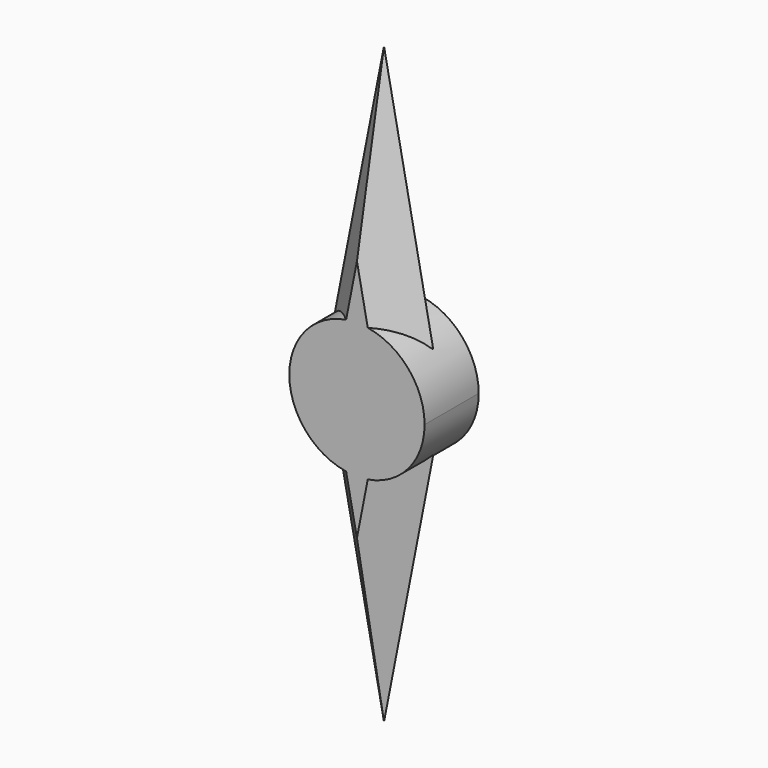
from build123d import *

# Parameters (mm, degrees)
F1_DEPTH = 12.7
F2_SIZE  = 6.34999


# Not quite as in the source:
# - a fillet or chamfer is up to 0.001 mm smaller than in the source, because OpenCascade refuses the exact size


with BuildPart() as f1:
    # F0 (on Front) → F1 (new body)
    with BuildSketch(Plane.XZ):
        with BuildLine():
            Line((0, 0), (12.7, 0))
            ThreePointArc((12.7, 0), (11.8071097568, 4.6778370206), (9.2539906785, 8.6979110436))
            ThreePointArc((9.2539906785, 8.6979110436), (5.0411570967, 11.6566176538), (0, 12.7))
            Line((0, 12.7), (0, 0))
        make_face()
        with BuildLine():
            ThreePointArc((9.2539906785, -8.6979110436), (11.8071097568, -4.6778370206), (12.7, 0))
            Line((12.7, 0), (0, 0))
            Line((0, 0), (0, -12.7))
            ThreePointArc((0, -12.7), (5.0411570967, -11.6566176538), (9.2539906785, -8.6979110436))
        make_face()
        with BuildLine():
            ThreePointArc((0, 12.7), (5.0411570967, 11.6566176538), (9.2539906785, 8.6979110436))
            Line((9.2539906785, 8.6979110436), (0, 55.8542348444))
            Line((0, 55.8542348444), (-9.2539906785, 8.6979110436))
            ThreePointArc((-9.2539906785, 8.6979110436), (-5.0411570967, 11.6566176538), (0, 12.7))
        make_face()
        with BuildLine():
            Line((0, -55.8542348444), (9.2539906785, -8.6979110436))
            ThreePointArc((9.2539906785, -8.6979110436), (5.0411570967, -11.6566176538), (0, -12.7))
            ThreePointArc((0, -12.7), (-5.0411570967, -11.6566176538), (-9.2539906785, -8.6979110436))
            Line((-9.2539906785, -8.6979110436), (0, -55.8542348444))
        make_face()
        with BuildLine():
            Line((-12.7, 0), (0, 0))
            Line((0, 0), (0, 12.7))
            ThreePointArc((0, 12.7), (-5.0411570967, 11.6566176538), (-9.2539906785, 8.6979110436))
            ThreePointArc((-9.2539906785, 8.6979110436), (-11.8071097568, 4.6778370206), (-12.7, 0))
        make_face()
        with BuildLine():
            Line((0, -12.7), (0, 0))
            Line((0, 0), (-12.7, 0))
            ThreePointArc((-12.7, 0), (-11.8071097568, -4.6778370206), (-9.2539906785, -8.6979110436))
            ThreePointArc((-9.2539906785, -8.6979110436), (-5.0411570967, -11.6566176538), (0, -12.7))
        make_face()
    extrude(amount=F1_DEPTH)

    # F2 (size 6.35 in the source; OpenCascade refuses exactly that, so slightly less here)
    f2_edges = [f1.edges().sort_by_distance(p)[0] for p in [
        (4.626995, -12.7, 32.276073),
        (4.626995, 0, 32.276073),
        (-4.626995, -12.7, 32.276073),
        (-4.626995, 0, 32.276073),
        (-4.626995, -12.7, -32.276073),
        (4.626995, -12.7, -32.276073),
        (-4.626995, 0, -32.276073),
        (4.626995, 0, -32.276073),
    ]]
    chamfer(f2_edges, length=F2_SIZE)


solid = f1.part
